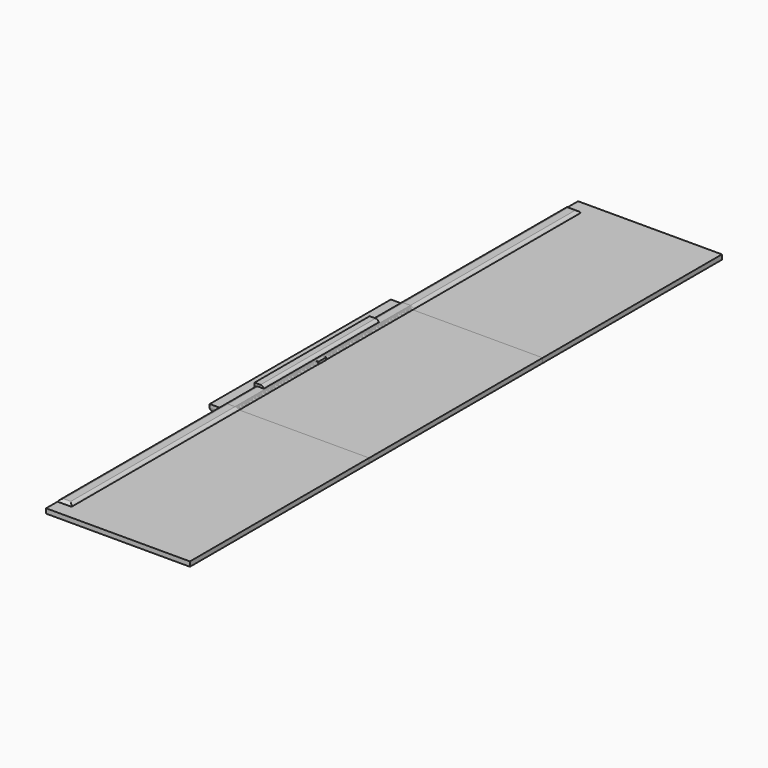
from build123d import *

# Parameters (mm, degrees)
F0_W          = 63.5
F0_H          = 19.05
F1_DEPTH      = 304.8
F2_R          = 9.525
F3_W          = 38.1
F3_H          = 19.05
F4_DEPTH      = 304.8
F5_R          = 9.525
F6_W          = 38.1
F6_H          = 19.05
F7_DEPTH      = 857.25
F8_R          = 9.525
F9_W          = 38.1
F9_H          = 19.05
F10_DEPTH     = 266.7
F11_R         = 9.525
F12_DEPTH     = 25.4
F13_W         = 25.4
F13_H         = 25.4
F14_DEPTH     = 193.675
F15_R         = 9.525
F17_D         = 6.35
F17_DEPTH     = 12.7
F17_TIP       = 1.9077324654
F19_D         = 6.35
F19_DEPTH     = 12.7
F19_TIP       = 1.9077324654
F20_T1_DEPTH  = 33.3375
F20_S5_W      = 9.525
F20_S5_H      = 9.525
F20_T6_DEPTH  = 9.525
F20_S11_W     = 9.525
F20_S11_H     = 9.525
F20_T12_DEPTH = 9.525
F21_W         = 387.35
F21_H         = 12.7
F22_DEPTH     = 279.4
F23_W         = 387.35
F23_H         = 12.7
F24_DEPTH     = 895.35
F25_W         = 387.35
F25_H         = 12.7
F26_DEPTH     = 292.1


# Not quite as in the source:
# - a fillet or chamfer that OpenCascade refuses, or shapes differently, is made with other operations: its cross-section is extruded or revolved along the edge and cut away or added


with BuildPart() as f1:
    # F0 (on Front) → F1 (new body, symmetric)
    with BuildSketch(Plane.XZ):
        Rectangle(F0_W, F0_H)
    extrude(amount=F1_DEPTH, both=True)

    # F2
    f2_edges = [f1.edges().sort_by_distance(p)[0] for p in [
        (31.75, 0, -9.525),
        (-31.75, 0, -9.525),
        (0, -304.8, -9.525),
        (0, 304.8, -9.525),
    ]]
    fillet(f2_edges, radius=F2_R)


with BuildPart() as f4:
    # F3 (on Front) → F4 (new body, symmetric)
    with BuildSketch(Plane.XZ):
        with Locations((19.05, 9.525)):
            Rectangle(F3_W, F3_H)
    extrude(amount=F4_DEPTH, both=True)

    # F5
    f5_edges = [f4.edges().sort_by_distance(p)[0] for p in [
        (38.1, 0, 19.05),
        (0, 0, 19.05),
        (19.05, -304.8, 19.05),
        (19.05, 304.8, 19.05),
    ]]
    fillet(f5_edges, radius=F5_R)

    # F20: fillet of radius 9.525 on 2 edges, made by hand

    # F20_s2 → F20_t1 (cut)
    with BuildSketch(Plane.XY.offset(-23.8125)):
        with BuildLine():
            ThreePointArc((28.575, -304.8), (35.3101920908, -302.0101920908), (38.1, -295.275))
            Line((38.1, -295.275), (38.1, -304.8))
            Line((38.1, -304.8), (28.575, -304.8))
        make_face()
        with BuildLine():
            ThreePointArc((28.575, 304.8), (35.3101920908, 302.0101920908), (38.1, 295.275))
            Line((38.1, 295.275), (38.1, 304.8))
            Line((38.1, 304.8), (28.575, 304.8))
        make_face()
    extrude(amount=F20_T1_DEPTH, mode=Mode.SUBTRACT)


with BuildPart() as f7:
    # F6 (on Front) → F7 (new body, symmetric)
    with BuildSketch(Plane.XZ):
        with Locations((19.05, 9.525)):
            Rectangle(F6_W, F6_H)
    extrude(amount=F7_DEPTH, both=True)

    # F8
    f8_edges = [f7.edges().sort_by_distance(p)[0] for p in [
        (38.1, 0, 19.05),
        (0, 0, 19.05),
        (19.05, -857.25, 19.05),
        (19.05, 857.25, 19.05),
    ]]
    fillet(f8_edges, radius=F8_R)


with BuildPart() as f10:
    # F9 (on Front) → F10 (new body, symmetric)
    with BuildSketch(Plane.XZ):
        with Locations((19.05, 9.525)):
            Rectangle(F9_W, F9_H)
    extrude(amount=F10_DEPTH, both=True)

    # F11
    f11_edges = [f10.edges().sort_by_distance(p)[0] for p in [
        (38.1, 0, 19.05),
        (0, 0, 19.05),
        (19.05, -266.7, 19.05),
        (19.05, 266.7, 19.05),
    ]]
    fillet(f11_edges, radius=F11_R)


with BuildPart() as f12:
    # F9 (on Front) → F12 (new body)
    with BuildSketch(Plane.XZ):
        with Locations((19.05, 9.525)):
            Rectangle(F9_W, F9_H)
    extrude(amount=F12_DEPTH)


with BuildPart() as f14:
    # F13 (on Front) → F14 (new body, symmetric)
    with BuildSketch(Plane.XZ):
        with Locations((12.7, 12.7)):
            Rectangle(F13_W, F13_H)
    extrude(amount=F14_DEPTH, both=True)

    # F15
    f15_edges = [f14.edges().sort_by_distance(p)[0] for p in [
        (25.4, 0, 25.4),
    ]]
    fillet(f15_edges, radius=F15_R)

    # F17
    with Locations(Plane(origin=(0, 0, 0), x_dir=(0, -1, 0), z_dir=(-1, 0, 0))):
        with Locations((-96.8375, 19.05), (0, 19.05), (96.8375, 19.05)):
            Hole(F17_D / 2, depth=F17_DEPTH)
            with Locations((0, 0, -(F17_DEPTH + F17_TIP / 2))):  # 118° drill point
                Cone(0, F17_D / 2, F17_TIP, mode=Mode.SUBTRACT)

    # F19
    with Locations(Plane(origin=(0, 0, 0), x_dir=(1, 0, 0), z_dir=(0, 0, -1))):
        with Locations((19.05, 96.8375), (19.05, 0), (19.05, -96.8375)):
            Hole(F19_D / 2, depth=F19_DEPTH)
            with Locations((0, 0, -(F19_DEPTH + F19_TIP / 2))):  # 118° drill point
                Cone(0, F19_D / 2, F19_TIP, mode=Mode.SUBTRACT)


with BuildPart() as f20_tool4:
    # F20_s5 → F20_t6 (new body)
    with BuildSketch(Plane.XZ.offset(-295.275)):
        with Locations((33.3375, 14.2875)):
            Rectangle(F20_S5_W, F20_S5_H)
    extrude(amount=-F20_T6_DEPTH)

    # F20_s7 → F20_t8 (revolve, cut)
    with BuildSketch(Plane(origin=(28.575, 295.275, 9.525), x_dir=(-0.7071067812, 0, -0.7071067812), z_dir=(0.7071067812, 0, -0.7071067812))):
        with BuildLine():
            ThreePointArc((0, -9.525), (9.525, 0), (0, 9.525))
            Line((0, 9.525), (0, -9.525))
        make_face()
    revolve(axis=Axis((28.575, 295.275, 9.525), (0, 1, 0)), mode=Mode.SUBTRACT)


with BuildPart() as f4_1:
    add(f4.part)

    # F20_t3: cut F20_tool4
    add(f20_tool4.part, mode=Mode.SUBTRACT)


with BuildPart() as f20_tool10:
    # F20_s11 → F20_t12 (new body)
    with BuildSketch(Plane.XZ.offset(295.275)):
        with Locations((33.3375, 14.2875)):
            Rectangle(F20_S11_W, F20_S11_H)
    extrude(amount=F20_T12_DEPTH)

    # F20_s13 → F20_t14 (revolve, cut)
    with BuildSketch(Plane(origin=(28.575, -295.275, 9.525), x_dir=(-0.7071067812, 0, -0.7071067812), z_dir=(-0.7071067812, 0, 0.7071067812))):
        with BuildLine():
            ThreePointArc((0, -9.525), (9.525, 0), (0, 9.525))
            Line((0, 9.525), (0, -9.525))
        make_face()
    revolve(axis=Axis((28.575, -295.275, 9.525), (0, -1, 0)), mode=Mode.SUBTRACT)


with BuildPart() as f4_2:
    add(f4_1.part)

    # F20_t9: cut F20_tool10
    add(f20_tool10.part, mode=Mode.SUBTRACT)


with BuildPart() as f22:
    # F21 (on Front) → F22 (new body, symmetric)
    with BuildSketch(Plane.XZ):
        with Locations((193.675, 6.35)):
            Rectangle(F21_W, F21_H)
    extrude(amount=F22_DEPTH, both=True)


with BuildPart() as f24:
    # F23 (on Front) → F24 (new body, symmetric)
    with BuildSketch(Plane.XZ):
        with Locations((193.675, 6.35)):
            Rectangle(F23_W, F23_H)
    extrude(amount=F24_DEPTH, both=True)


with BuildPart() as f26:
    # F25 (on Front) → F26 (new body, symmetric)
    with BuildSketch(Plane.XZ):
        with Locations((193.675, 6.35)):
            Rectangle(F25_W, F25_H)
    extrude(amount=F26_DEPTH, both=True)


solid = Compound([f1.part, f7.part, f10.part, f12.part, f14.part, f4_2.part, f22.part, f24.part, f26.part])
